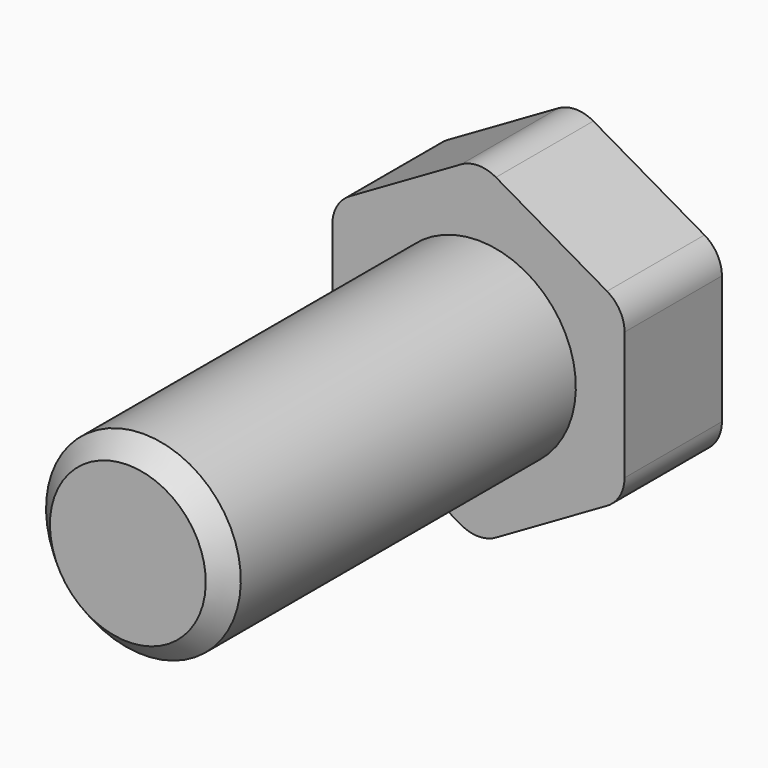
from build123d import *

# Parameters (mm, degrees)
F2_R     = 25.1475
F3_DEPTH = 25


# Not quite as in the source:
# - a feature names something its author has since deleted; it is built from what else it names


with BuildPart() as f1:
    # F0 (on Right) → F1 (revolve)
    with BuildSketch(Plane.YZ):
        Polygon((0, 25.1475), (0, 10), (-43, 10), (-45, 8), (-45, 0), (12.5, 0), (12.5, 25.1475), align=None)
    revolve(axis=Axis((0, -16.25, 0), (0, -1, 0)))

    # F2 (on face) → F3 (cut)
    with BuildSketch(Plane(origin=(0, 12.5, 0), x_dir=(-1, 0, 0), z_dir=(0, 1, 0))):
        Circle(F2_R)
        with BuildLine():
            ThreePointArc((1.7954303246, -16.2839158944), (0, -16.765), (-1.7954303246, -16.2839158944))
            Line((-1.7954303246, -16.2839158944), (-13.2045696754, -9.6968462191))
            ThreePointArc((-13.2045696754, -9.6968462191), (-14.5189158944, -8.3825), (-15, -6.5870696754))
            Line((-15, -6.5870696754), (-15, 6.5870696754))
            ThreePointArc((-15, 6.5870696754), (-14.5189158944, 8.3825), (-13.2045696754, 9.6968462191))
            Line((-13.2045696754, 9.6968462191), (-1.7954303246, 16.2839158944))
            ThreePointArc((-1.7954303246, 16.2839158944), (0, 16.765), (1.7954303246, 16.2839158944))
            Line((1.7954303246, 16.2839158944), (13.2045696754, 9.6968462191))
            ThreePointArc((13.2045696754, 9.6968462191), (14.5189158944, 8.3825), (15, 6.5870696754))
            Line((15, 6.5870696754), (15, -6.5870696754))
            ThreePointArc((15, -6.5870696754), (14.5189158944, -8.3825), (13.2045696754, -9.6968462191))
            Line((13.2045696754, -9.6968462191), (1.7954303246, -16.2839158944))
        make_face(mode=Mode.SUBTRACT)
    extrude(amount=-F3_DEPTH, mode=Mode.SUBTRACT)


solid = f1.part
